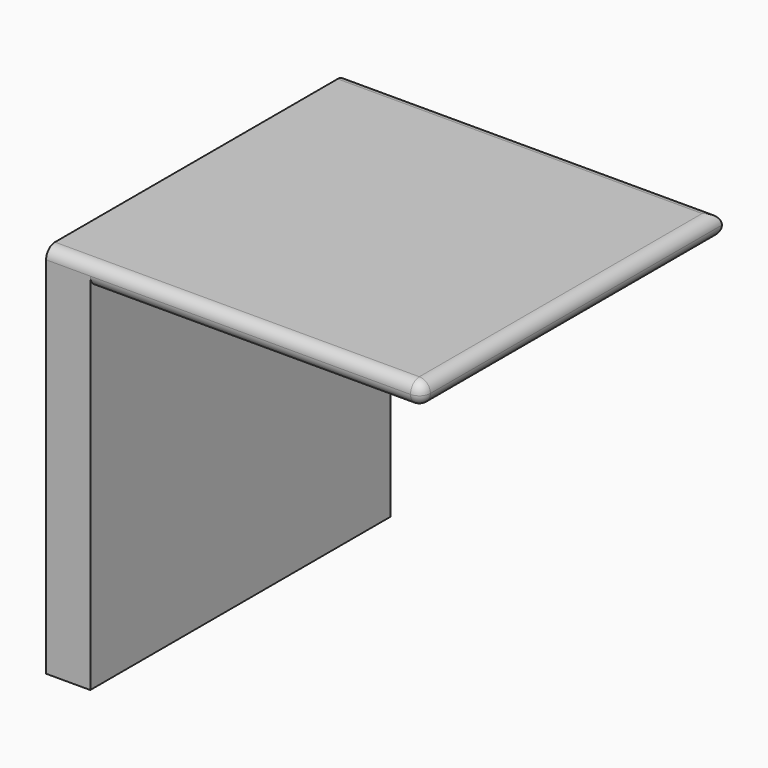
from build123d import *

# Parameters (mm, degrees)
F0_W     = 431.8
F0_H     = 25.4
F1_DEPTH = 431.8
F0_H_2   = 406.4
F2_DEPTH = 50.8
F3_R     = 12.69999


# Not quite as in the source:
# - a fillet or chamfer is up to 0.001 mm smaller than in the source, because OpenCascade refuses the exact size


with BuildPart() as f1:
    # F0 (on Right) → F1 (new body)
    with BuildSketch(Plane.YZ):
        with Locations((0, 203.2)):
            Rectangle(F0_W, F0_H)
    extrude(amount=F1_DEPTH)

    # F0 (on Right) → F2 (join)
    with BuildSketch(Plane.YZ):
        with Locations((0, -12.7)):
            Rectangle(F0_W, F0_H_2)
    extrude(amount=F2_DEPTH)

    # F3 (radius 12.7 in the source; OpenCascade refuses exactly that, so slightly less here)
    f3_edges = [f1.edges().sort_by_distance(p)[0] for p in [
        (431.8, 0, 190.5),
        (431.8, -215.9, 203.2),
        (241.3, -215.9, 190.5),
        (215.9, -215.9, 215.9),
        (431.8, 0, 215.9),
        (215.9, 215.9, 215.9),
        (241.3, 215.9, 190.5),
    ]]
    fillet(f3_edges, radius=F3_R)


solid = f1.part
